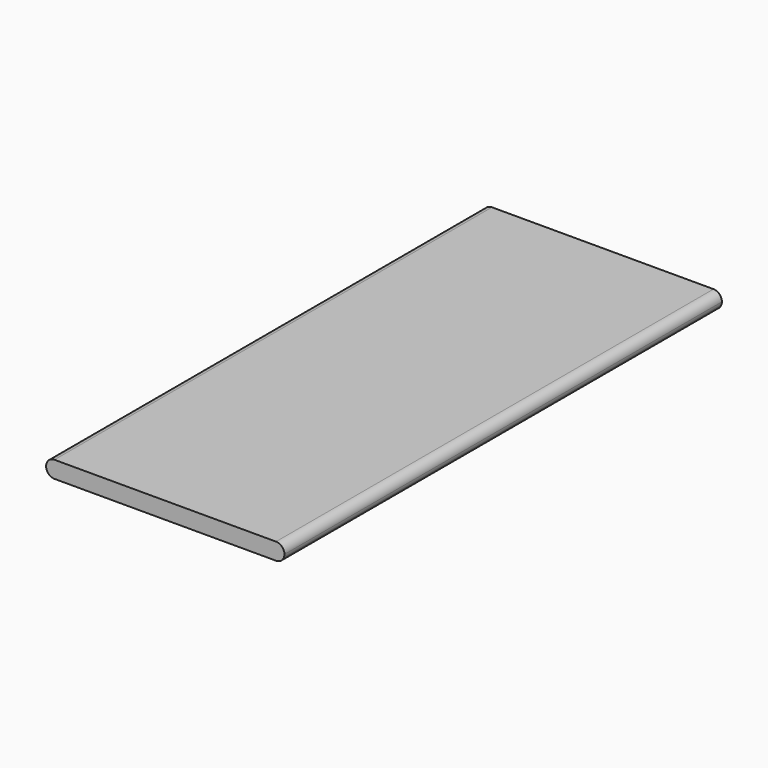
from build123d import *

# Parameters (mm, degrees)
F0_W     = 17
F0_H     = 1.2
F1_DEPTH = 39
F2_R     = 0.59999


# Not quite as in the source:
# - a fillet or chamfer is up to 0.001 mm smaller than in the source, because OpenCascade refuses the exact size


with BuildPart() as f1:
    # F0 (on Front) → F1 (new body)
    with BuildSketch(Plane.XZ):
        Rectangle(F0_W, F0_H)
    extrude(amount=F1_DEPTH)

    # F2 (radius 0.6 in the source; OpenCascade refuses exactly that, so slightly less here)
    f2_edges = [f1.edges().sort_by_distance(p)[0] for p in [
        (8.5, -19.5, 0.6),
        (-8.5, -19.5, 0.6),
        (8.5, -19.5, -0.6),
        (-8.5, -19.5, -0.6),
    ]]
    fillet(f2_edges, radius=F2_R)


solid = f1.part
